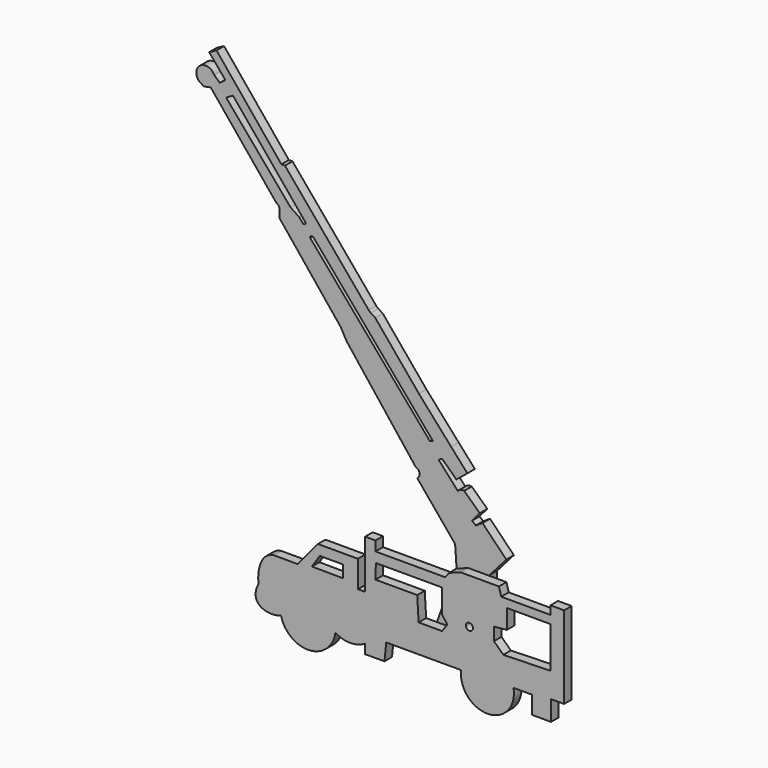
from build123d import *

# Parameters (mm, degrees)
F1_DEPTH  = 12.7
F2_DEPTH  = 12.7
F4_DEPTH  = 12.7
F5_R      = 4.7625
F6_DEPTH  = 25.4010001
F7_R      = 23.9856001161
F7_R_2    = 2.2430927124
F7_R_3    = 2.7133749082
F8_DEPTH  = 12.7
F9_DEPTH  = 6.35
F10_R     = 3.4789562926
F11_DEPTH = 12.7
F13_DEPTH = 6.35
F14_R     = 3.4245437789
F15_DEPTH = 11.43


with BuildPart() as f1:
    # F0 (on Front) → F1 (new body)
    with BuildSketch(Plane.XZ):
        with BuildLine():
            Line((-148.623675108, -251.2744069099), (-176.1702746153, -284.0453386307))
            Line((-176.1702746153, -284.0453386307), (-208.0560326576, -283.9412093163))
            add(Edge.make_bspline(
                [(-208.0560326576, -283.9412093163), (-227.9891073704, -286.6129279137), (-230.4546684027, -312.9496574402), (-228.6865264177, -324.4474232197)],
                knots=[0, 0, 0, 0, 45.4573496541, 45.4573496541, 45.4573496541, 45.4573496541], degree=3))
            add(Edge.make_bspline(
                [(-198.3723400416, -352.3083863628), (-215.0639295578, -359.0107560158), (-243.1187182665, -351.9504368305), (-228.6865264177, -324.4474232197)],
                knots=[0, 0, 0, 0, 41.1726020906, 41.1726020906, 41.1726020906, 41.1726020906], degree=3))
            ThreePointArc((-198.3723400416, -352.3083863628), (-160.258361309, -381.2026055114), (-125.0308901072, -348.8517701626))
            ThreePointArc((-125.0308901072, -348.8517701626), (-105.029374361, -354.5426889584), (-85.0278586149, -348.8517701626))
            Line((-85.0278586149, -348.8517701626), (-85.0278586149, -361.4313304424))
            Line((-85.0278586149, -361.4313304424), (-58.8623546064, -361.4313304424))
            Line((-58.8623546064, -361.4313304424), (-56.485068053, -338.1886482239))
            Line((-56.485068053, -338.1886482239), (44.4399528205, -338.1886482239))
            ThreePointArc((44.4399528205, -338.1886482239), (80.9287484221, -378.4247975339), (115.2061969042, -336.288869381))
            Line((115.2061969042, -336.288869381), (139.9031430483, -336.288869381))
            Line((139.9031430483, -336.288869381), (139.9031430483, -360.2734208107))
            Line((139.9031430483, -360.2734208107), (165.7874435186, -360.2734208107))
            Line((165.7874435186, -360.2734208107), (165.7874435186, -333.2017660141))
            Line((165.7874435186, -333.2017660141), (183.4268522694, -333.2017660141))
            Line((183.4268522694, -333.2017660141), (183.4268522694, -222.0655083656))
            Line((183.4268522694, -222.0655083656), (165.0750339031, -222.0655083656))
            Line((165.0750339031, -222.0655083656), (165.0750339031, -233.4640920162))
            Line((165.0750339031, -233.4640920162), (98.5832586884, -233.4640920162))
            Line((98.5832586884, -233.4640920162), (95.4961329699, -222.3029732704))
            Line((95.4961329699, -222.3029732704), (44.2024804652, -222.3029732704))
            Line((44.2024804652, -222.3029732704), (28.2919500023, -228.0022650957))
            Line((28.2919500023, -228.0022650957), (22.8301230818, -234.8889261484))
            Line((22.8301230818, -234.8889261484), (-70.9707736969, -234.8889261484))
            Line((-70.9707736969, -234.8889261484), (-70.9707736969, -221.8280285597))
            Line((-70.9707736969, -221.8280285597), (-84.9815458059, -221.8280285597))
            Line((-84.9815458059, -221.8280285597), (-84.9815458059, -287.3699367046))
            Line((-84.9815458059, -287.3699367046), (-94.7178378701, -287.3699367046))
            Line((-94.7178378701, -287.3699367046), (-94.7178378701, -251.2744069099))
            Line((-94.7178378701, -251.2744069099), (-148.623675108, -251.2744069099))
        make_face()
        Polygon((-114.7156432271, -280.9221148491), (-156.7313969135, -280.6705236435), (-146.1645662785, -264.568656683), (-114.7156432271, -264.568656683), align=None, mode=Mode.SUBTRACT)
        Polygon((-14.6902352571, -268.3722674847), (-70.9707736969, -268.3722674847), (-70.4958364367, -248.4247386456), (18.7931228429, -248.4247386456), (18.7931228429, -280.7207405567), (25.9172413498, -290.2195751667), (18.7931228429, -300.1933395863), (-12.7904703841, -300.1933395863), align=None, mode=Mode.SUBTRACT)
        Polygon((106.1413660645, -244.3902790546), (165.1672422886, -244.3902790546), (165.1672422886, -299.8195886612), (101.4869958162, -301.5120923519), (88.7932553887, -289.4530594349), (88.7932553887, -272.1049487591), (106.1413660645, -270.4124450684), align=None, mode=Mode.SUBTRACT)
    extrude(amount=F1_DEPTH)


with BuildPart() as f2:
    # F0 (on Front) → F2 (new body)
    with BuildSketch(Plane.XZ):
        with BuildLine():
            Line((-295.5166399479, 281.8103348285), (-305.5061101913, 276.5258848667))
            Line((-305.5061101913, 276.5258848667), (-283.6389839649, 250.5414783955))
            Line((-283.6389839649, 250.5414783955), (-291.035681963, 244.7137534618))
            Line((-291.035681963, 244.7137534618), (-298.6565232277, 251.6621649265))
            ThreePointArc((-298.6565232277, 251.6621649265), (-317.3317448363, 256.8458672977), (-319.0535008907, 237.5411987305))
            Line((-319.0535008907, 237.5411987305), (-312.7775192261, 233.5066348314))
            Line((-312.7775192261, 233.5066348314), (-303.3635318279, 235.2997809649))
            Line((-303.3635318279, 235.2997809649), (-214.9053066969, 127.0917654037))
            ThreePointArc((-214.9053066969, 127.0917654037), (-211.8448364528, 124.6300222289), (-210.2648764849, 121.0341379046))
            Line((-210.2648764849, 121.0341379046), (-210.2648764849, 115.3032779694))
            Line((-210.2648764849, 115.3032779694), (-210.9978944063, 112.1046543121))
            Line((-210.9978944063, 112.1046543121), (-210.3981524706, 110.0388765335))
            Line((-210.3981524706, 110.0388765335), (-128.0732154846, 7.9876165837))
            Line((-128.0732154846, 7.9876165837), (-120.2282384038, -6.245427765))
            Line((-120.2282384038, -6.245427765), (-26.6702454537, -125.7143169641))
            ThreePointArc((-26.6702454537, -125.7143169641), (-21.6440973232, -131.2160222268), (-24.8771067709, -137.9300802946))
            Line((-24.8771067709, -137.9300802946), (24.2424178869, -197.158113122))
            Line((24.2424178869, -197.158113122), (26.252258569, -200.0142037868))
            Line((26.252258569, -200.0142037868), (28.1563196331, -226.6710549593))
            Line((28.1563196331, -226.6710549593), (43.7061488628, -221.1704403162))
            Line((43.7061488628, -221.1704403162), (72.9017406702, -221.1704403162))
            Line((72.9017406702, -221.1704403162), (95.327347517, -195.5713927746))
            Line((95.327347517, -195.5713927746), (63.1984695792, -162.7169549465))
            Line((63.1984695792, -162.7169549465), (54.1040604179, -168.5415186318))
            Line((54.1040604179, -168.5415186318), (49.1489805281, -164.3407642841))
            Line((49.1489805281, -164.3407642841), (59.4652481377, -152.1720141172))
            Line((59.4652481377, -152.1720141172), (38.4076610208, -132.4471831322))
            ThreePointArc((38.4076610208, -132.4471831322), (33.7606719727, -132.8333793183), (29.8113636672, -135.3126168251))
            Line((29.8113636672, -135.3126168251), (4.2190486565, -107.0035099983))
            ThreePointArc((4.2190486565, -107.0035099983), (6.5261180021, -105.1937439525), (9.4023244455, -104.6234294772))
            Line((9.4023244455, -104.6234294772), (27.9669146985, -122.4475502968))
            Line((27.9669146985, -122.4475502968), (42.7852012217, -110.303811729))
            Line((42.7852012217, -110.303811729), (20.9132172167, -85.8959406614))
            Line((20.9132172167, -85.8959406614), (-22.5137639791, -37.0802134275))
            Line((-22.5137639791, -37.0802134275), (-81.5027877688, 34.0543538332))
            Line((-81.5027877688, 34.0543538332), (-87.4395519495, 37.6164130867))
            Line((-87.4395519495, 37.6164130867), (-90.2892053127, 40.2285903692))
            Line((-90.2892053127, 40.2285903692), (-203.2371610403, 175.0263720751))
            Line((-203.2371610403, 175.0263720751), (-208.1030905247, 175.0263720751))
            Line((-208.1030905247, 175.0263720751), (-295.5166399479, 281.8103348285))
        make_face()
        Polygon((-168.6714142561, 102.803952992), (-165.0979667902, 102.8078794479), (-3.4802661536, -87.2205462625), (-7.7417450957, -88.5988175869), (-169.2591309547, 100.2851948142), align=None, mode=Mode.SUBTRACT)
        with BuildLine():
            Line((-195.6214308739, 127.8545707464), (-282.5182676315, 230.0269752741))
            Line((-282.5182676315, 230.0269752741), (-273.3284235001, 235.4063987732))
            Line((-273.3284235001, 235.4063987732), (-176.0522127151, 117.3583641648))
            ThreePointArc((-176.0522127151, 117.3583641648), (-176.3456741259, 114.3162934557), (-179.3877448351, 114.6097548664))
            Line((-179.3877448351, 114.6097548664), (-184.0328445244, 120.2467434421))
            Line((-184.0328445244, 120.2467434421), (-195.6214308739, 127.8545707464))
        make_face(mode=Mode.SUBTRACT)
    extrude(amount=-F2_DEPTH)

    # F3 (on face) → F4 (join)
    with BuildSketch(Plane(origin=(0, 12.7, 0), x_dir=(-1, 0, 0), z_dir=(0, 1, 0))):
        with BuildLine():
            Line((-72.9017406702, -221.1704403162), (-72.9017406702, -344.3099721307))
            ThreePointArc((-72.9017406702, -344.3099721307), (-29.2351651474, -340.9298417021), (1.8566996307, -310.0835932394))
            Line((1.8566996307, -310.0835932394), (-28.1563196331, -226.6710549593))
            Line((-28.1563196331, -226.6710549593), (-43.7061488628, -221.1704403162))
            Line((-43.7061488628, -221.1704403162), (-72.9017406702, -221.1704403162))
        make_face()
    extrude(amount=-F4_DEPTH)


with BuildPart() as f6_tool:
    # F5 (on face) → F6 (new body, through all)
    with BuildSketch(Plane(origin=(0, 12.7, 0), x_dir=(-1, 0, 0), z_dir=(0, 1, 0))):
        with Locations((-55.6685438016, -283.1931419963)):
            Circle(F5_R)
    extrude(amount=-F6_DEPTH)


with BuildPart() as f1_1:
    add(f1.part)

    # F6: cut by f6_tool
    add(f6_tool.part, mode=Mode.SUBTRACT)

    # F7 (on face) → F9 (cut)
    with BuildSketch(Plane.XZ):
        with Locations((-123.6301138997, -313.1083548069)):
            Circle(F7_R_3)
    extrude(amount=F9_DEPTH, mode=Mode.SUBTRACT)


with BuildPart() as f2_1:
    add(f2.part)

    # F6: cut by f6_tool
    add(f6_tool.part, mode=Mode.SUBTRACT)

    # F10 (on face) → F11 (cut)
    with BuildSketch(Plane(origin=(0, 12.7, 0), x_dir=(-1, 0, 0), z_dir=(0, 1, 0))):
        with Locations((-21.347252652, -320.2348649502)):
            Circle(F10_R)
    extrude(amount=-F11_DEPTH, mode=Mode.SUBTRACT)


with BuildPart() as f8:
    # F7 (on face) → F8 (new body)
    with BuildSketch(Plane.XZ):
        with Locations((-123.6301138997, -313.1083548069)):
            Circle(F7_R)
        with Locations((-142.6267887667, -311.6839798568)):
            Circle(F7_R_2, mode=Mode.SUBTRACT)
        with Locations((-123.6301138997, -313.1083548069)):
            Circle(F7_R_3, mode=Mode.SUBTRACT)
    extrude(amount=-F8_DEPTH)


with BuildPart() as f13:
    # F12 (on face) → F13 (new body)
    with BuildSketch(Plane(origin=(0, 12.7, 0), x_dir=(-1, 0, 0), z_dir=(0, 1, 0))):
        with BuildLine():
            Line((142.4434353917, -309.4483934781), (-19.7932642209, -317.1222684711))
            ThreePointArc((-19.7932642209, -317.1222684711), (-24.8211974287, -320.4215319649), (-19.4686739604, -323.1630177784))
            Line((-19.4686739604, -323.1630177784), (142.8272785425, -313.918094618))
            ThreePointArc((142.8272785425, -313.918094618), (144.8616557614, -311.4920568708), (142.4434353917, -309.4483934781))
        make_face()
    extrude(amount=F13_DEPTH)

    # F14 (on face) → F15 (join)
    with BuildSketch(Plane.XZ.offset(-12.7)):
        with Locations((21.347252652, -320.2348649502)):
            Circle(F14_R)
        with BuildLine():
            Line((-142.4434353917, -309.4483934781), (-140.8724086278, -309.52270381))
            ThreePointArc((-140.8724086278, -309.52270381), (-145.4067035153, -311.5389356845), (-141.1068547789, -314.0160957403))
            Line((-141.1068547789, -314.0160957403), (-142.8272785425, -313.918094618))
            ThreePointArc((-142.8272785425, -313.918094618), (-144.8616557614, -311.4920568708), (-142.4434353917, -309.4483934781))
        make_face()
        with BuildLine():
            ThreePointArc((-141.1068547789, -314.0160957403), (-140.1793413113, -313.0102395504), (-139.8430926946, -311.6839798568))
            ThreePointArc((-139.8430926946, -311.6839798568), (-140.1135612677, -310.4870457065), (-140.8724086278, -309.52270381))
            Line((-140.8724086278, -309.52270381), (-142.4434353917, -309.4483934781))
            ThreePointArc((-142.4434353917, -309.4483934781), (-144.8616557614, -311.4920568708), (-142.8272785425, -313.918094618))
            Line((-142.8272785425, -313.918094618), (-141.1068547789, -314.0160957403))
        make_face()
    extrude(amount=F15_DEPTH)


solid = Compound([f1_1.part, f2_1.part, f8.part, f13.part])
